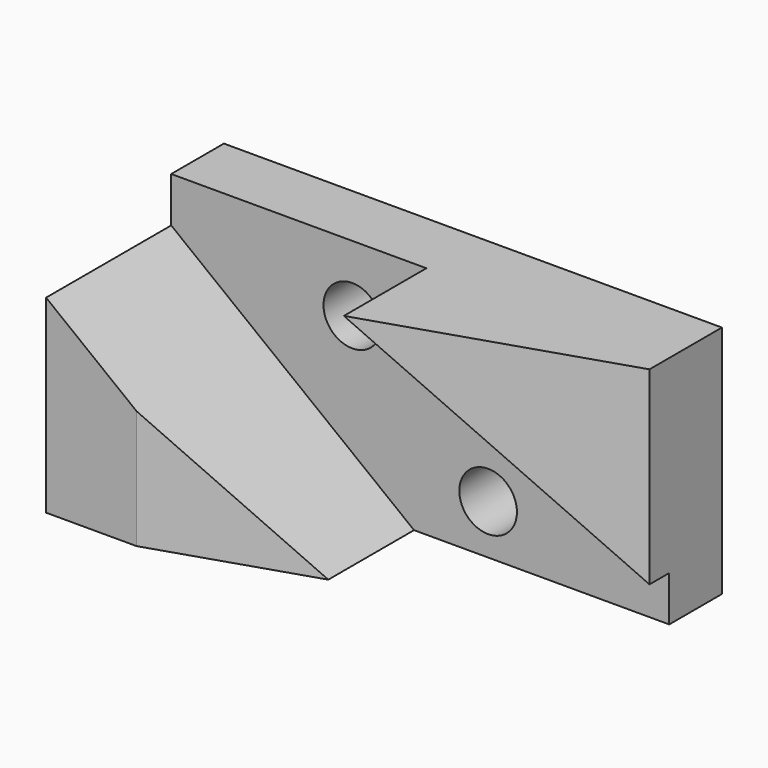
from build123d import *

# Parameters (mm, degrees)
F0_R     = 7
F1_DEPTH = 16
F2_DEPTH = 54
F4_DEPTH = 57.001
F6_DEPTH = 57.001


with BuildPart() as f1:
    # F0 (on Front) → F1 (new body)
    with BuildSketch(Plane.XZ):
        Polygon((0, 46), (59, 0), (121, 0), (121, 11), (62, 57), (0, 57), align=None)
        with Locations((77, 12)):
            Circle(F0_R, mode=Mode.SUBTRACT)
        with Locations((44, 41)):
            Circle(F0_R, mode=Mode.SUBTRACT)
    extrude(amount=F1_DEPTH)

    # F0 (on Front) → F2 (join)
    with BuildSketch(Plane.XZ):
        Polygon((0, 46), (0, 0), (59, 0), align=None)
        Polygon((62, 57), (121, 11), (121, 57), align=None)
    extrude(amount=F2_DEPTH)

    # F3 (on face) → F4 (cut, through all)
    with BuildSketch(Plane.XY.offset(57)):
        Polygon((121, -54), (121, -22), (62, -41.0707070707), (62, -54), align=None)
    extrude(amount=-F4_DEPTH, mode=Mode.SUBTRACT)

    # F5 (on face) → F6 (cut, through all)
    with BuildSketch(Plane(origin=(0, 0, 0), x_dir=(1, 0, 0), z_dir=(0, 0, -1))):
        Polygon((59, 54), (22, 54), (59, 42.0404040404), align=None)
    extrude(amount=-F6_DEPTH, mode=Mode.SUBTRACT)


solid = f1.part
